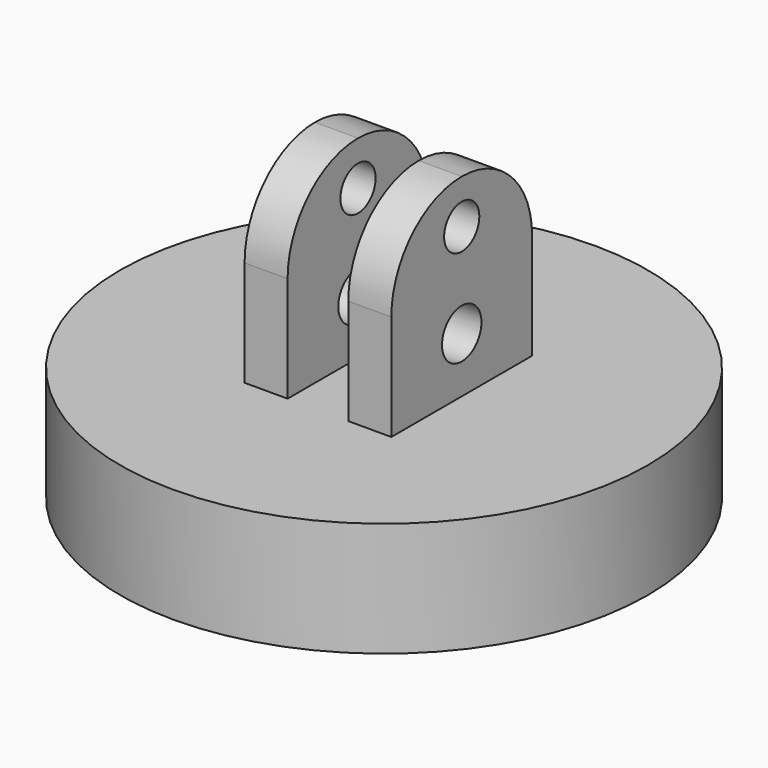
from build123d import *

# Parameters (mm, degrees)
F0_R     = 38.1
F1_DEPTH = 16.51
F2_W     = 6.20888776
F2_H     = 25.4
F2_W_2   = 6.2088776
F3_DEPTH = 27.94
F4_R     = 12.69999
F5_R     = 3.556
F5_R_2   = 3.175
F6_DEPTH = 49.319129452


# Not quite as in the source:
# - a fillet or chamfer is up to 0.001 mm smaller than in the source, because OpenCascade refuses the exact size


with BuildPart() as f1:
    # F0 (on Top) → F1 (new body)
    with BuildSketch(Plane.XY):
        Circle(F0_R)
    extrude(amount=F1_DEPTH)

    # F2 (on face) → F3 (join)
    with BuildSketch(Plane.XY.offset(16.51)):
        with Locations((-6.858192028, 0)):
            Rectangle(F2_W, F2_H)
        with Locations((8.113690652, 0)):
            Rectangle(F2_W_2, F2_H)
    extrude(amount=F3_DEPTH)

    # F4 (radius 12.7 in the source; OpenCascade refuses exactly that, so slightly less here)
    f4_edges = [f1.edges().sort_by_distance(p)[0] for p in [
        (-6.858192, 12.7, 44.45),
        (-6.858192, -12.7, 44.45),
        (8.113691, -12.7, 44.45),
        (8.113691, 12.7, 44.45),
    ]]
    fillet(f4_edges, radius=F4_R)

    # F5 (on face) → F6 (cut, through all)
    with BuildSketch(Plane.YZ.offset(11.218129452)):
        with Locations((0, 24.4883745909)):
            Circle(F5_R)
        with Locations((0, 38.0773745909)):
            Circle(F5_R_2)
    extrude(amount=-F6_DEPTH, mode=Mode.SUBTRACT)


solid = f1.part
